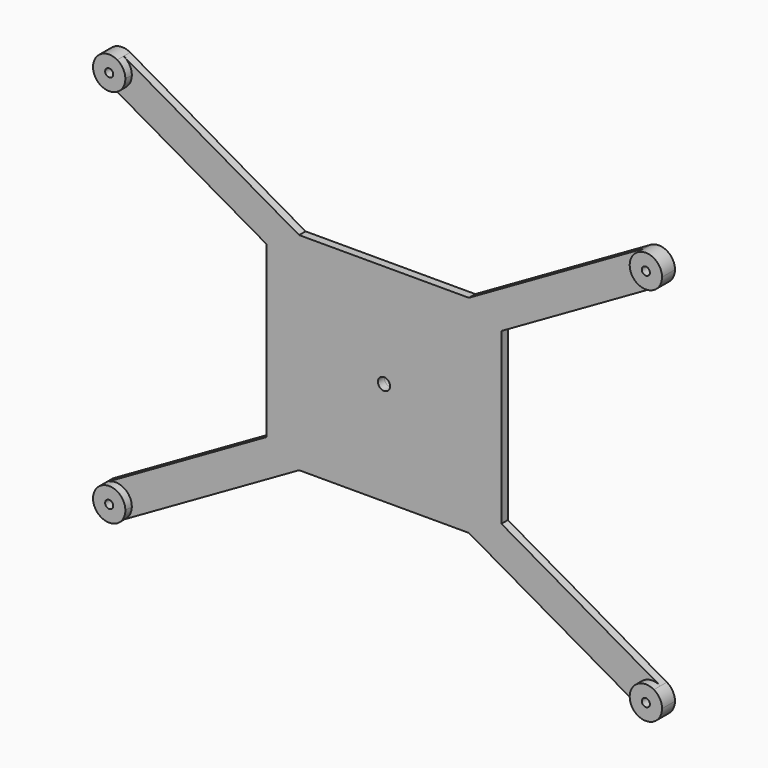
from build123d import *

# Parameters (mm, degrees)
F1_DEPTH = 5
F0_R     = 2.5
F2_DEPTH = 10
F3_ANGLE = 180
F4_DEPTH = 45


# Not quite as in the source:
# - a feature names something its author has since deleted; it is built from what else it names


with BuildPart() as f1:
    # F0 (on Front) → F1 (new body)
    with BuildSketch(Plane.XZ):
        with BuildLine():
            Line((52.5, 64.0237609195), (-52.5, 64.0237609195))
            Line((-52.5, 64.0237609195), (-161.030379156, 126.1777225507))
            ThreePointArc((-161.030379156, 126.1777225507), (-157.3485201139, 122.5151665755), (-156, 117.5))
            ThreePointArc((-156, 117.5), (-160.9848334245, 108.8485201139), (-170.969620844, 108.8222774493))
            Line((-170.969620844, 108.8222774493), (-72.6222594518, 52.5))
            Line((-72.6222594518, 52.5), (-72.6222594518, -52.5))
            Line((-72.6222594518, -52.5), (-170.969620844, -108.8222774493))
            ThreePointArc((-170.969620844, -108.8222774493), (-160.9848334245, -108.8485201139), (-156, -117.5))
            ThreePointArc((-156, -117.5), (-157.3485201139, -122.5151665755), (-161.030379156, -126.1777225507))
            Line((-161.030379156, -126.1777225507), (-52.5, -64.0237609195))
            Line((-52.5, -64.0237609195), (52.5, -64.0237609195))
            Line((52.5, -64.0237609195), (161.030379156, -126.1777225507))
            ThreePointArc((161.030379156, -126.1777225507), (157.3222774493, -112.530379156), (170.969620844, -108.8222774493))
            Line((170.969620844, -108.8222774493), (72.6222594518, -52.5))
            Line((72.6222594518, -52.5), (72.6222594518, 52.5))
            Line((72.6222594518, 52.5), (170.969620844, 108.8222774493))
            ThreePointArc((170.969620844, 108.8222774493), (157.3222774493, 112.530379156), (161.030379156, 126.1777225507))
            Line((161.030379156, 126.1777225507), (52.5, 64.0237609195))
        make_face()
        with BuildLine():
            Line((45, 0), (3.75, 0))
            ThreePointArc((3.75, 0), (0, -3.75), (-3.75, 0))
            Line((-3.75, 0), (-45, 0))
            ThreePointArc((-45, 0), (0, 45), (45, 0))
        make_face(mode=Mode.SUBTRACT)
        with BuildLine():
            ThreePointArc((-3.75, 0), (0, 3.75), (3.75, 0))
            Line((3.75, 0), (45, 0))
            ThreePointArc((45, 0), (0, 45), (-45, 0))
            Line((-45, 0), (-3.75, 0))
        make_face()
    extrude(amount=F1_DEPTH)

    # F0 (on Front) → F2 (join)
    with BuildSketch(Plane.XZ):
        with BuildLine():
            ThreePointArc((-156, 117.5), (-157.3485201139, 122.5151665755), (-161.030379156, 126.1777225507))
            ThreePointArc((-161.030379156, 126.1777225507), (-174.6777225507, 122.469620844), (-170.969620844, 108.8222774493))
            ThreePointArc((-170.969620844, 108.8222774493), (-160.9848334245, 108.8485201139), (-156, 117.5))
        make_face()
        with Locations((-166, 117.5)):
            Circle(F0_R, mode=Mode.SUBTRACT)
        with BuildLine():
            ThreePointArc((176, -117.5), (174.6514798861, -112.4848334245), (170.969620844, -108.8222774493))
            ThreePointArc((170.969620844, -108.8222774493), (157.3222774493, -112.530379156), (161.030379156, -126.1777225507))
            ThreePointArc((161.030379156, -126.1777225507), (171.0151665755, -126.1514798861), (176, -117.5))
        make_face()
        with Locations((166, -117.5)):
            Circle(F0_R, mode=Mode.SUBTRACT)
        with BuildLine():
            ThreePointArc((176, 117.5), (171.0151665755, 126.1514798861), (161.030379156, 126.1777225507))
            ThreePointArc((161.030379156, 126.1777225507), (157.3222774493, 112.530379156), (170.969620844, 108.8222774493))
            ThreePointArc((170.969620844, 108.8222774493), (174.6514798861, 112.4848334245), (176, 117.5))
        make_face()
        with Locations((166, 117.5)):
            Circle(F0_R, mode=Mode.SUBTRACT)
        with BuildLine():
            ThreePointArc((-156, -117.5), (-160.9848334245, -108.8485201139), (-170.969620844, -108.8222774493))
            ThreePointArc((-170.969620844, -108.8222774493), (-174.6777225507, -122.469620844), (-161.030379156, -126.1777225507))
            ThreePointArc((-161.030379156, -126.1777225507), (-157.3485201139, -122.5151665755), (-156, -117.5))
        make_face()
        with Locations((-166, -117.5)):
            Circle(F0_R, mode=Mode.SUBTRACT)
    extrude(amount=F2_DEPTH)

    # F0 (on Front) → F3 (revolve)
    with BuildSketch(Plane.XZ):
        with BuildLine():
            ThreePointArc((-3.75, 0), (0, 3.75), (3.75, 0))
            Line((3.75, 0), (45, 0))
            ThreePointArc((45, 0), (0, 45), (-45, 0))
            Line((-45, 0), (-3.75, 0))
        make_face()
    revolve(axis=Axis((0, 0, 0), (-1, 0, 0)), revolution_arc=F3_ANGLE)

    # F0 (on Front) → F4 (cut)
    with BuildSketch(Plane.XZ):
        with BuildLine():
            ThreePointArc((-3.75, 0), (0, -3.75), (3.75, 0))
            Line((3.75, 0), (-3.75, 0))
        make_face()
        with BuildLine():
            Line((-3.75, 0), (3.75, 0))
            ThreePointArc((3.75, 0), (0, 3.75), (-3.75, 0))
        make_face()
    extrude(amount=-F4_DEPTH, mode=Mode.SUBTRACT)


solid = f1.part
